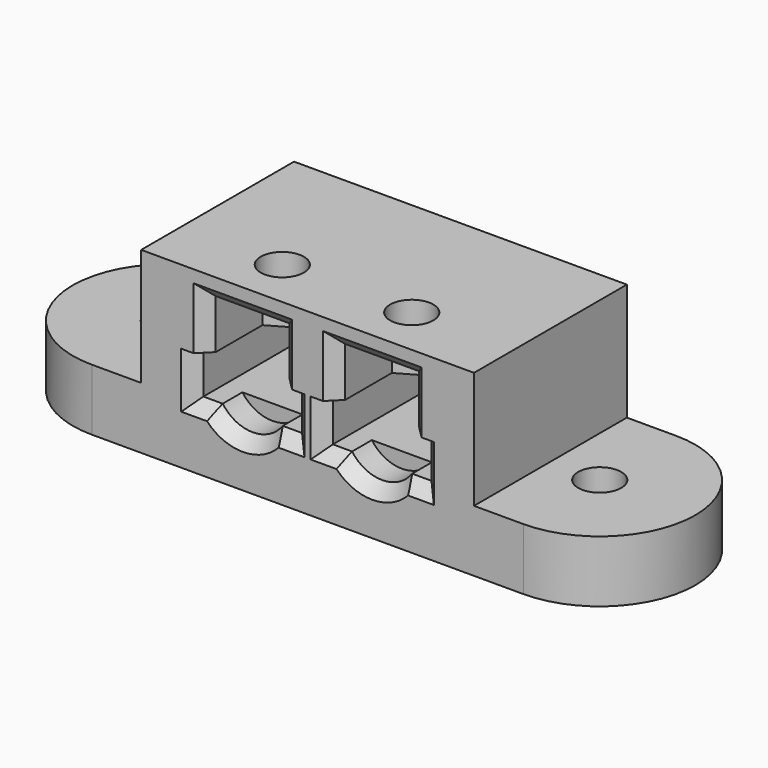
from build123d import *

# Parameters (mm, degrees)
F1_DEPTH      = 3.5
F0_W          = 1.25
F0_H          = 11.5
F2_W          = 21
F2_H          = 11.5
F3_DEPTH      = 2
F4_W          = 27
F4_H          = 14.5
F4_W_2        = 21
F4_H_2        = 5.5
F5_DEPTH      = 11.5
F5_DEPTH_BACK = 4
F6_R          = 1.75
F7_DEPTH      = 25
F9_DEPTH      = 4
F10_R         = 3
F11_DEPTH     = 3
F12_SIZE      = 0.9999
F13_R         = 1.75
F14_DEPTH     = 5


# Not quite as in the source:
# - a fillet or chamfer is up to 0.001 mm smaller than in the source, because OpenCascade refuses the exact size


with BuildPart() as f1:
    # F0 (on Top) → F1 (new body)
    with BuildSketch(Plane.XY):
        Polygon((1.25, 0), (0, 0), (-1.25, 0), (-1.25, -11.5), (0, -11.5), (1.25, -11.5), align=None)
    extrude(amount=F1_DEPTH)



with BuildPart() as f1b:
    # F0 (on Top) → F1, piece 2 (new body)
    with BuildSketch(Plane.XY):
        with Locations((-9.875, -5.75)):
            Rectangle(F0_W, F0_H)
    extrude(amount=F1_DEPTH)


with BuildPart() as f1c:
    # F0 (on Top) → F1, piece 3 (new body)
    with BuildSketch(Plane.XY):
        with Locations((9.875, -5.75)):
            Rectangle(F0_W, F0_H)
    extrude(amount=F1_DEPTH)


with BuildPart() as f1_1:
    add(f1.part)

    add(f1b.part)  # F3 merges F1b

    add(f1c.part)  # F3 merges F1c
    # F2 (on Top) → F3 (join)
    with BuildSketch(Plane.XY):
        with Locations((0, -5.75)):
            Rectangle(F2_W, F2_H)
    extrude(amount=-F3_DEPTH)

    # F4 (on Front) → F5 (join, two sides)
    with BuildSketch(Plane.XZ) as f5_sk:
        with Locations((0, 2.25)):
            Rectangle(F4_W, F4_H)
        with Locations((0, 0.75)):
            Rectangle(F4_W_2, F4_H_2, mode=Mode.SUBTRACT)
    extrude(amount=F5_DEPTH)
    extrude(f5_sk.sketch, amount=-F5_DEPTH_BACK)

    # F6 (on face) → F7 (cut)
    with BuildSketch(Plane.XY):
        with Locations((5.25, -7.5)):
            Circle(F6_R)
        with Locations((-5.25, -7.5)):
            Circle(F6_R)
    extrude(amount=F7_DEPTH, mode=Mode.SUBTRACT)

    # F8 (on face) → F9 (cut)
    with BuildSketch(Plane(origin=(0, 0, 3.5), x_dir=(1, 0, 0), z_dir=(0, 0, -1))):
        Polygon((2.25, 5.7679491924), (5.25, 4.0358983849), (8.25, 5.7679491924), (8.25, 9.2320508076), (5.25, 10.9641016151), (2.25, 9.2320508076), align=None)
        Polygon((2.25, 21.0246167397), (2.25, 9.2320508076), (5.25, 10.9641016151), (8.25, 9.2320508076), (8.25, 21.0246167397), align=None)
        Polygon((-2.25, 21.0246167397), (-8.25, 21.0246167397), (-8.25, 9.2320508076), (-8.25, 5.7679491924), (-5.25, 4.0358983849), (-2.25, 5.7679491924), (-2.25, 9.2320508076), align=None)
    extrude(amount=-F9_DEPTH, mode=Mode.SUBTRACT)

    # F10 (on face) → F11 (cut)
    with BuildSketch(Plane.XZ.offset(11.5)):
        with Locations((5.25, 1.75)):
            Circle(F10_R)
        with Locations((-5.25, 1.75)):
            Circle(F10_R)
    extrude(amount=-F11_DEPTH, mode=Mode.SUBTRACT)

    # F12 (size 1 in the source; OpenCascade refuses exactly that, so slightly less here)
    f12_edges = [f1_1.edges().sort_by_distance(p)[0] for p in [
        (-1.25, -11.5, 1.75),
        (-9.25, -11.5, 1.75),
        (-2.031651, -11.5, 0),
        (-8.468349, -11.5, 0),
        (2.031651, -11.5, 0),
        (1.25, -11.5, 1.75),
        (5.25, -11.5, -1.25),
        (8.468349, -11.5, 0),
        (9.25, -11.5, 1.75),
        (-5.25, -11.5, -1.25),
        (-8.25, -11.5, 5.5),
        (-5.25, -11.5, 7.5),
        (-2.25, -11.5, 5.5),
        (2.25, -11.5, 5.5),
        (5.25, -11.5, 7.5),
        (8.25, -11.5, 5.5),
    ]]
    chamfer(f12_edges, length=F12_SIZE)

    # F13 (on face) → F14 (join)
    with BuildSketch(Plane(origin=(0, 0, -5), x_dir=(1, 0, 0), z_dir=(0, 0, -1))):
        with BuildLine():
            Line((13.5, -4), (17.5, -4))
            ThreePointArc((17.5, -4), (25.25, 3.75), (17.5, 11.5))
            Line((17.5, 11.5), (13.5, 11.5))
            Line((13.5, 11.5000000001), (13.5, -4))
        make_face()
        with Locations((17.5, 3.75)):
            Circle(F13_R, mode=Mode.SUBTRACT)
        with BuildLine():
            ThreePointArc((-17.5, 11.5), (-25.25, 3.75), (-17.5, -4))
            Line((-17.5, -4), (-13.5, -4))
            Line((-13.5, -4), (-13.5, 11.5000000001))
            Line((-13.5, 11.5), (-17.5, 11.5))
        make_face()
        with Locations((-17.5, 3.75)):
            Circle(F13_R, mode=Mode.SUBTRACT)
    extrude(amount=-F14_DEPTH)


solid = f1_1.part
